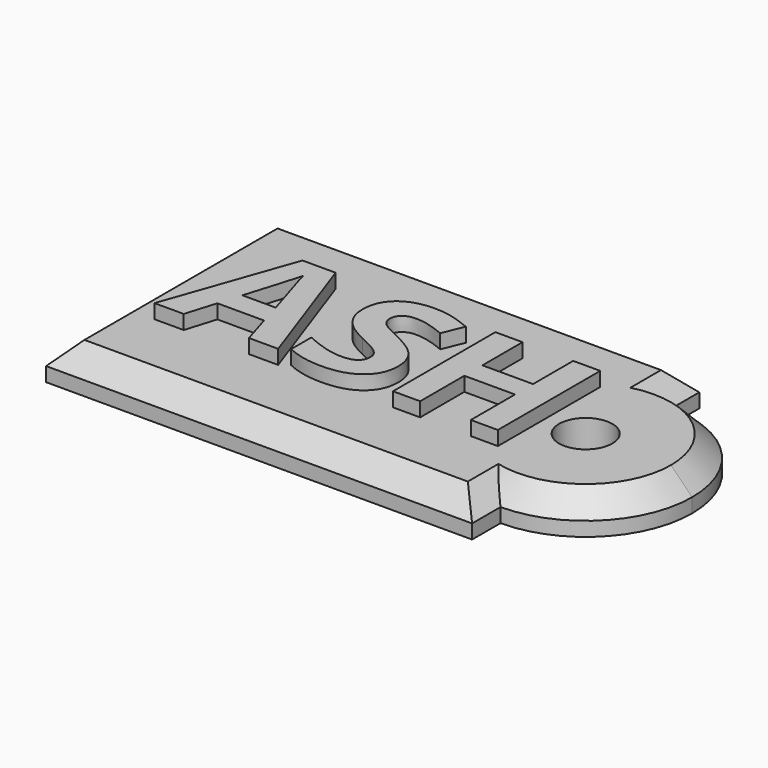
from build123d import *

# Parameters (mm, degrees)
F0_W         = 76.2
F0_H         = 50.8
F1_DEPTH     = 6.35
F3_DEPTH     = 6.35
F4_TEXT_SIZE = 32.0631163708
F5_DEPTH     = 2.54
F7_D         = 9.525
F8_SIZE      = 3.81


# Not quite as in the source:
# - Text() gives the source's letters only with a copy of the font that has no kerning and outlines rounded to 1/6400 em; it was checked with that copy


with BuildPart() as f1:
    # F0 (on Top) → F1 (new body)
    with BuildSketch(Plane.XY):
        with Locations((38.1, 25.4)):
            Rectangle(F0_W, F0_H)
    extrude(amount=F1_DEPTH)

    # F2 (on face) → F3 (join)
    with BuildSketch(Plane.XY.offset(6.35)):
        with BuildLine():
            ThreePointArc((76.2, 6.35), (89.6703841816, 11.9296158184), (95.25, 25.4))
            ThreePointArc((95.25, 25.4), (89.6703841816, 38.8703841816), (76.2, 44.45))
            Line((76.2, 44.45), (76.2, 6.35))
        make_face()
    extrude(amount=-F3_DEPTH)

    # F4 (on face) → F5 (join)
    with BuildSketch(Plane.XY.offset(6.35)):
        with Locations((7.5486134758, 14.7995814061)):
            Text('ASH', F4_TEXT_SIZE, font='Open Sans', font_style=FontStyle.BOLD, text_align=(TextAlign.LEFT, TextAlign.BOTTOM))
    extrude(amount=F5_DEPTH)

    # F7 (through all)
    with Locations(Plane.XY.offset(6.35)):
        with Locations((76.2, 25.4)):
            Hole(F7_D / 2)

    # F8
    f8_edges = [f1.edges().sort_by_distance(p)[0] for p in [
        (0, 25.4, 6.35),
        (38.1, 0, 6.35),
        (38.1, 50.8, 6.35),
        (76.2, 47.625, 6.35),
        (95.25, 25.4, 6.35),
        (76.2, 3.175, 6.35),
    ]]
    chamfer(f8_edges, length=F8_SIZE)


solid = f1.part
